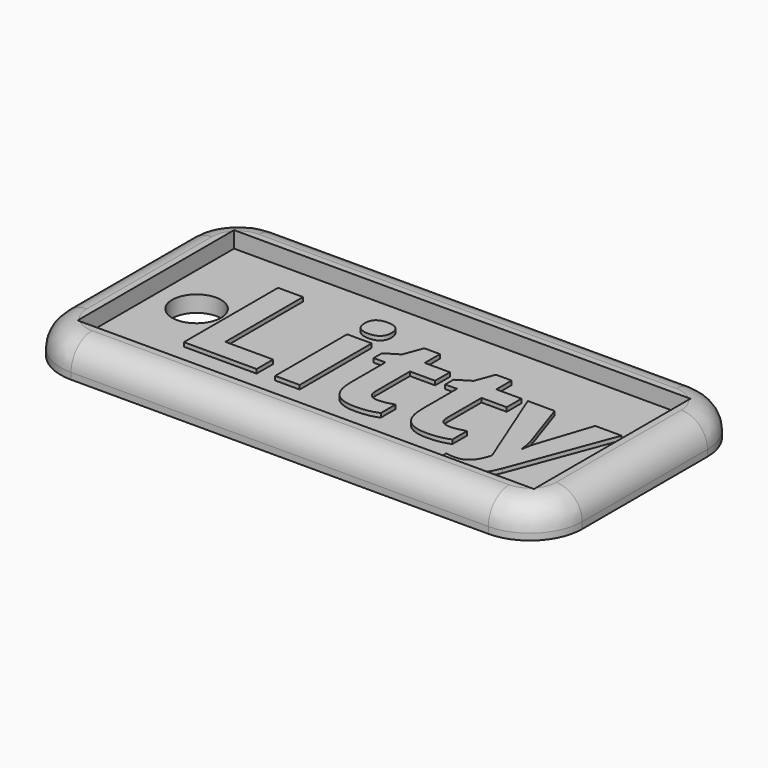
from build123d import *

# Parameters (mm, degrees)
F0_W         = 44.45
F0_H         = 19.05
F0_R         = 2.38125
F1_DEPTH     = 1.5875
F0_W_2       = 50.8
F0_H_2       = 25.4
F2_DEPTH     = 3.175
F3_R         = 5.08
F4_T1_DEPTH  = 40.64
F4_T3_DEPTH  = 15.24
F4_T6_ANGLE  = 90
F4_T8_ANGLE  = 90
F4_T10_ANGLE = 90
F4_T12_ANGLE = 90
F5_TEXT_SIZE = 16.0621829919
F6_DEPTH     = 0.396875


# Not quite as in the source:
# - a fillet or chamfer that OpenCascade refuses, or shapes differently, is made with other operations: its cross-section is extruded or revolved along the edge and cut away or added
# - Text() gives the source's letters only with a copy of the font that has no kerning and outlines rounded to 1/6400 em; it was checked with that copy


with BuildPart() as f1:
    # F0 (on Top) → F1 (new body)
    with BuildSketch(Plane.XY):
        with Locations((25.4, 12.7)):
            Rectangle(F0_W, F0_H)
        with Locations((7.14375, 12.7)):
            Circle(F0_R, mode=Mode.SUBTRACT)
    extrude(amount=F1_DEPTH)

    # F0 (on Top) → F2 (join)
    with BuildSketch(Plane.XY):
        with Locations((25.4, 12.7)):
            Rectangle(F0_W_2, F0_H_2)
        with Locations((25.4, 12.7)):
            Rectangle(F0_W, F0_H, mode=Mode.SUBTRACT)
    extrude(amount=F2_DEPTH)

    # F3
    f3_edges = [f1.edges().sort_by_distance(p)[0] for p in [
        (50.8, 25.4, 1.5875),
        (50.8, 0, 1.5875),
        (0, 0, 1.5875),
        (0, 25.4, 1.5875),
    ]]
    fillet(f3_edges, radius=F3_R)

    # F4: fillet of radius 2.54 on 8 edges, made by hand

    # F4_s2 → F4_t1 (cut)
    with BuildSketch(Plane.YZ.offset(5.08)):
        with BuildLine():
            ThreePointArc((0, 0.635), (0.7439487758, 2.4310512242), (2.54, 3.175))
            Line((2.54, 3.175), (0, 3.175))
            Line((0, 3.175), (0, 0.635))
        make_face()
        with BuildLine():
            ThreePointArc((25.4, 0.635), (24.6560512242, 2.4310512242), (22.86, 3.175))
            Line((22.86, 3.175), (25.4, 3.175))
            Line((25.4, 3.175), (25.4, 0.635))
        make_face()
    extrude(amount=F4_T1_DEPTH, mode=Mode.SUBTRACT)

    # F4_s4 → F4_t3 (cut)
    with BuildSketch(Plane.XZ.offset(-20.32)):
        with BuildLine():
            ThreePointArc((0, 0.635), (0.7439487758, 2.4310512242), (2.54, 3.175))
            Line((2.54, 3.175), (0, 3.175))
            Line((0, 3.175), (0, 0.635))
        make_face()
        with BuildLine():
            ThreePointArc((50.8, 0.635), (50.0560512242, 2.4310512242), (48.26, 3.175))
            Line((48.26, 3.175), (50.8, 3.175))
            Line((50.8, 3.175), (50.8, 0.635))
        make_face()
    extrude(amount=F4_T3_DEPTH, mode=Mode.SUBTRACT)

    # F4_s5 → F4_t6 (revolve, cut)
    with BuildSketch(Plane.XZ.offset(-20.32)):
        with BuildLine():
            ThreePointArc((0, 0.635), (0.7439487758, 2.4310512242), (2.54, 3.175))
            Line((2.54, 3.175), (0, 3.175))
            Line((0, 3.175), (0, 0.635))
        make_face()
    revolve(axis=Axis((5.08, 20.32, 3.175), (0, 0, -1)), revolution_arc=F4_T6_ANGLE, mode=Mode.SUBTRACT)

    # F4_s7 → F4_t8 (revolve, cut)
    with BuildSketch(Plane.XZ.offset(-5.08)):
        with BuildLine():
            ThreePointArc((0, 0.635), (0.7439487758, 2.4310512242), (2.54, 3.175))
            Line((2.54, 3.175), (0, 3.175))
            Line((0, 3.175), (0, 0.635))
        make_face()
    revolve(axis=Axis((5.08, 5.08, 3.175), (0, 0, 1)), revolution_arc=F4_T8_ANGLE, mode=Mode.SUBTRACT)

    # F4_s9 → F4_t10 (revolve, cut)
    with BuildSketch(Plane.XZ.offset(-20.32)):
        with BuildLine():
            ThreePointArc((50.8, 0.635), (50.0560512242, 2.4310512242), (48.26, 3.175))
            Line((48.26, 3.175), (50.8, 3.175))
            Line((50.8, 3.175), (50.8, 0.635))
        make_face()
    revolve(axis=Axis((45.72, 20.32, 3.175), (0, 0, 1)), revolution_arc=F4_T10_ANGLE, mode=Mode.SUBTRACT)

    # F4_s11 → F4_t12 (revolve, cut)
    with BuildSketch(Plane.YZ.offset(45.72)):
        with BuildLine():
            ThreePointArc((0, 0.635), (0.7439487758, 2.4310512242), (2.54, 3.175))
            Line((2.54, 3.175), (0, 3.175))
            Line((0, 3.175), (0, 0.635))
        make_face()
    revolve(axis=Axis((45.72, 5.08, 3.175), (0, 0, 1)), revolution_arc=F4_T12_ANGLE, mode=Mode.SUBTRACT)

    # F5 (on face) → F6 (join)
    with BuildSketch(Plane.XY.offset(1.5875)):
        with Locations((8.8529778564, 7.2166371978)):
            Text('Litty', F5_TEXT_SIZE, font='Open Sans', font_style=FontStyle.BOLD, text_align=(TextAlign.LEFT, TextAlign.BOTTOM))
    extrude(amount=F6_DEPTH)


solid = f1.part
